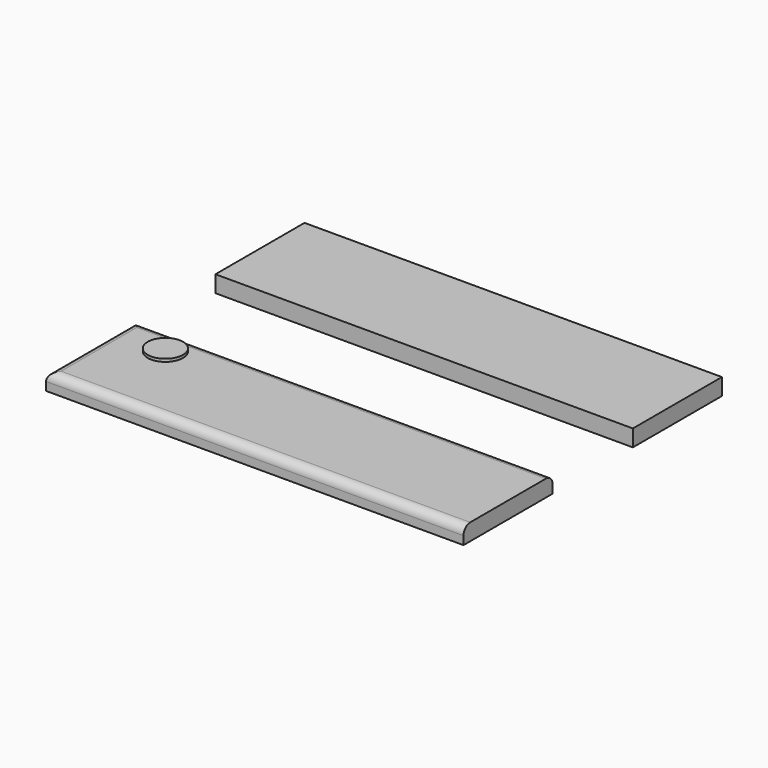
from build123d import *

# Parameters (mm, degrees)
F0_W        = 150
F0_H        = 40
F1_DEPTH    = 6
F2_W        = 150
F2_H        = 40
F3_DEPTH    = 6
F4_R        = 6.35
F5_DEPTH    = 1
F6_W        = 35
F6_H        = 10
F6_W_2      = 32.5
F7_DEPTH    = 3.5
F8_T1_DEPTH = 165
F8_T3_DEPTH = 55
F9_W        = 32.5
F9_H        = 10
F9_W_2      = 35
F10_DEPTH   = 3.5


# Not quite as in the source:
# - a fillet or chamfer that OpenCascade refuses, or shapes differently, is made with other operations: its cross-section is extruded or revolved along the edge and cut away or added


with BuildPart() as f1:
    # F0 (on Top) → F1 (new body)
    with BuildSketch(Plane.XY):
        Rectangle(F0_W, F0_H)
    extrude(amount=F1_DEPTH)

    # F9 (on face) → F10 (cut)
    with BuildSketch(Plane(origin=(0, 0, 0), x_dir=(1, 0, 0), z_dir=(0, 0, -1))):
        with Locations((55.625, -12.5)):
            Rectangle(F9_W, F9_H)
        with Locations((19.375, -12.5)):
            Rectangle(F9_W_2, F9_H)
        with Locations((55.625, 0)):
            Rectangle(F9_W, F9_H)
        with Locations((19.375, 0)):
            Rectangle(F9_W_2, F9_H)
        with Locations((55.625, 12.5)):
            Rectangle(F9_W, F9_H)
        with Locations((-18.125, -12.5)):
            Rectangle(F9_W_2, F9_H)
        with Locations((-55.625, -12.5)):
            Rectangle(F9_W_2, F9_H)
        with Locations((-55.625, 0)):
            Rectangle(F9_W_2, F9_H)
        with Locations((-55.625, 12.5)):
            Rectangle(F9_W_2, F9_H)
        with Locations((-18.125, 12.5)):
            Rectangle(F9_W_2, F9_H)
        with Locations((-18.125, 0)):
            Rectangle(F9_W_2, F9_H)
        with Locations((19.375, 12.5)):
            Rectangle(F9_W_2, F9_H)
    extrude(amount=-F10_DEPTH, mode=Mode.SUBTRACT)


with BuildPart() as f3:
    # F2 (on Top) → F3 (new body)
    with BuildSketch(Plane.XY):
        with Locations((0, -76.0728493333)):
            Rectangle(F2_W, F2_H)
    extrude(amount=F3_DEPTH)

    # F4 (on face) → F5 (join)
    with BuildSketch(Plane.XY.offset(6)):
        with Locations((-56.65, -65.4228493333)):
            Circle(F4_R)
    extrude(amount=F5_DEPTH)

    # F6 (on face) → F7 (cut)
    with BuildSketch(Plane(origin=(0, 0, 0), x_dir=(1, 0, 0), z_dir=(0, 0, -1))):
        with Locations((-55, 88.5728493333)):
            Rectangle(F6_W, F6_H)
        with Locations((-17.5, 88.5728493333)):
            Rectangle(F6_W, F6_H)
        with Locations((-17.5, 76.0728493333)):
            Rectangle(F6_W, F6_H)
        with Locations((-55, 76.0728493333)):
            Rectangle(F6_W, F6_H)
        with Locations((-55, 63.5728493333)):
            Rectangle(F6_W, F6_H)
        with Locations((20, 63.5728493333)):
            Rectangle(F6_W, F6_H)
        with Locations((20, 76.0728493333)):
            Rectangle(F6_W, F6_H)
        with Locations((20, 88.5728493333)):
            Rectangle(F6_W, F6_H)
        with Locations((-17.5, 63.5728493333)):
            Rectangle(F6_W, F6_H)
        with Locations((56.25, 88.5728493333)):
            Rectangle(F6_W_2, F6_H)
        with Locations((56.25, 76.0728493333)):
            Rectangle(F6_W_2, F6_H)
        with Locations((56.25, 63.5728493333)):
            Rectangle(F6_W_2, F6_H)
    extrude(amount=-F7_DEPTH, mode=Mode.SUBTRACT)

    # F8: fillet of radius 3 on 3 edges, made by hand

    # F8_s2 → F8_t1 (cut)
    with BuildSketch(Plane.YZ.offset(-82.5)):
        with BuildLine():
            ThreePointArc((-56.0728493333, 3), (-56.9515289897, 5.1213203436), (-59.0728493333, 6))
            Line((-59.0728493333, 6), (-56.0728493333, 6))
            Line((-56.0728493333, 6), (-56.0728493333, 3))
        make_face()
        with BuildLine():
            ThreePointArc((-96.0728493333, 3), (-95.1941696768, 5.1213203436), (-93.0728493333, 6))
            Line((-93.0728493333, 6), (-96.0728493333, 6))
            Line((-96.0728493333, 6), (-96.0728493333, 3))
        make_face()
    extrude(amount=F8_T1_DEPTH, mode=Mode.SUBTRACT)

    # F8_s4 → F8_t3 (cut)
    with BuildSketch(Plane.XZ.offset(48.5728493333)):
        with BuildLine():
            ThreePointArc((-72, 6), (-74.1213203436, 5.1213203436), (-75, 3))
            Line((-75, 3), (-75, 6))
            Line((-75, 6), (-72, 6))
        make_face()
    extrude(amount=F8_T3_DEPTH, mode=Mode.SUBTRACT)


solid = Compound([f1.part, f3.part])
